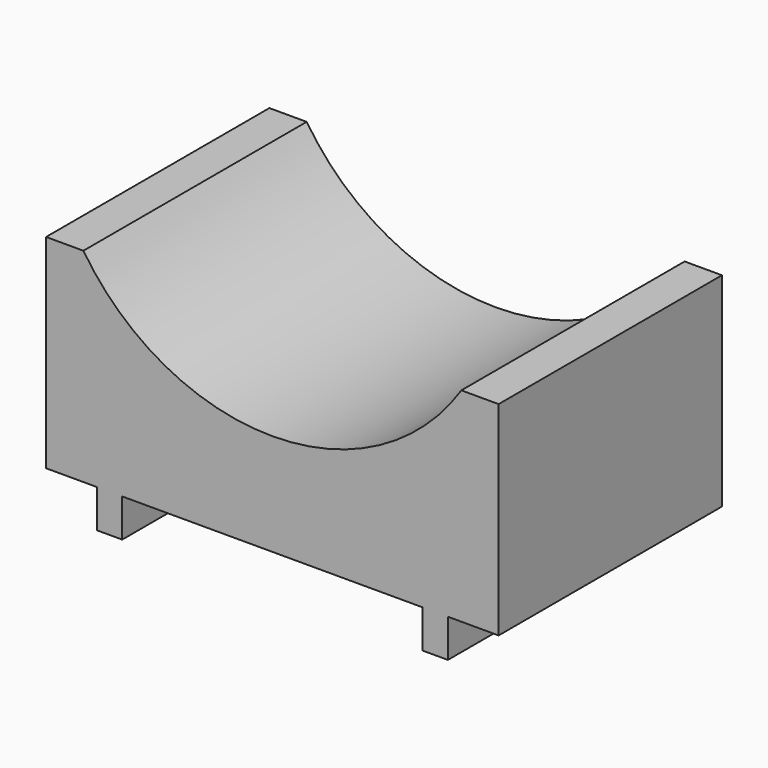
from build123d import *

# Parameters (mm, degrees)
F1_DEPTH = 220


# Not quite as in the source:
# - the program builds the solid bodies; features that only make, move or delete a surface that nothing else refers to are left out


with BuildPart() as f1:
    # F0 (on Front) → F1 (new body)
    with BuildSketch(Plane.XZ):
        with BuildLine():
            Line((-178.3572353468, 80.260755906), (-178.3572353468, -80.260755906))
            Line((-178.3572353468, -80.260755906), (-138.3572353468, -80.260755906))
            Line((-138.3572353468, -80.260755906), (-138.3572353468, -110.260755906))
            Line((-138.3572353468, -110.260755906), (-118.3572353468, -110.260755906))
            Line((-118.3572353468, -110.260755906), (-118.3572353468, -80.260755906))
            Line((-118.3572353468, -80.260755906), (118.3572353468, -80.260755906))
            Line((118.3572353468, -80.260755906), (118.3572353468, -110.260755906))
            Line((118.3572353468, -110.260755906), (138.3572353468, -110.260755906))
            Line((138.3572353468, -110.260755906), (138.3572353468, -80.260755906))
            Line((138.3572353468, -80.260755906), (178.3572353468, -80.260755906))
            Line((178.3572353468, -80.260755906), (178.3572353468, 80.260755906))
            Line((178.3572353468, 80.260755906), (148.9576588225, 80.260755906))
            ThreePointArc((148.9576588225, 80.260755906), (0, 0), (-148.9576588225, 80.260755906))
            Line((-148.9576588225, 80.260755906), (-178.3572353468, 80.260755906))
        make_face()
    extrude(amount=F1_DEPTH)


solid = f1.part
